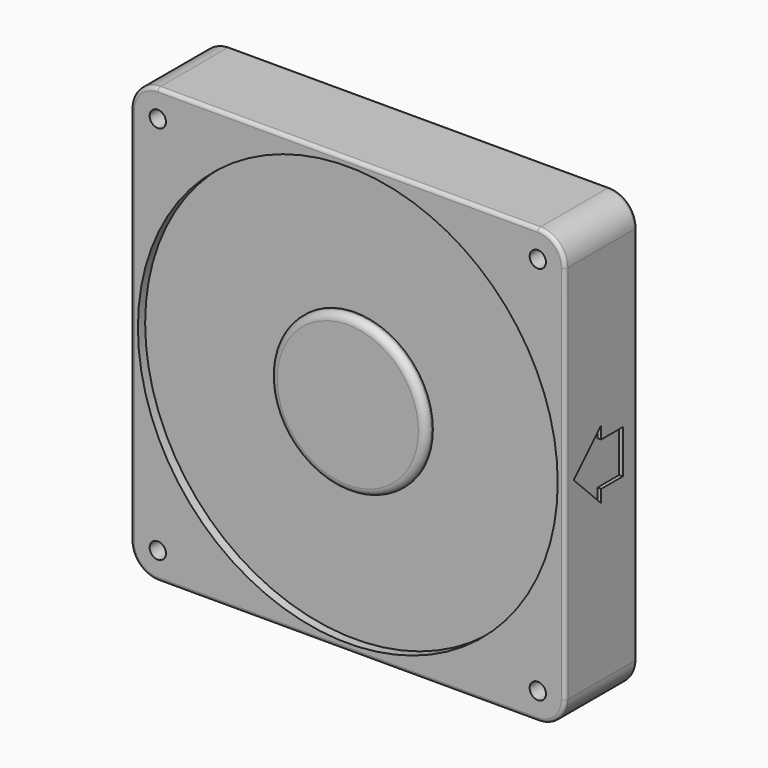
from build123d import *

# Parameters (mm, degrees)
F0_R      = 58
F1_DEPTH  = 12.5
F0_R_2    = 21.5
F2_DEPTH  = 10
F3_R      = 2
F4_R      = 1
F6_D      = 4.5
F8_DEPTH  = 1
F10_DEPTH = 1


with BuildPart() as f1:
    # F0 (on Front) → F1 (new body, symmetric)
    with BuildSketch(Plane.XZ):
        with BuildLine():
            Line((52.5, 60), (-52.5, 60))
            ThreePointArc((-52.5, 60), (-57.8033008589, 57.8033008589), (-60, 52.5))
            Line((-60, 52.5), (-60, -52.5))
            ThreePointArc((-60, -52.5), (-57.8033008589, -57.8033008589), (-52.5, -60))
            Line((-52.5, -60), (52.5, -60))
            ThreePointArc((52.5, -60), (57.8033008589, -57.8033008589), (60, -52.5))
            Line((60, -52.5), (60, 52.5))
            ThreePointArc((60, 52.5), (57.8033008589, 57.8033008589), (52.5, 60))
        make_face()
        Circle(F0_R, mode=Mode.SUBTRACT)
    extrude(amount=F1_DEPTH, both=True)

    # F4
    f4_edges = [f1.edges().sort_by_distance(p)[0] for p in [
        (-60, -12.5, 0),
        (-57.803301, -12.5, -57.803301),
        (0, -12.5, -60),
        (57.803301, -12.5, -57.803301),
        (60, -12.5, 0),
        (57.803301, -12.5, 57.803301),
        (0, -12.5, 60),
        (-57.803301, -12.5, 57.803301),
        (-57.803301, 12.5, -57.803301),
        (0, 12.5, -60),
        (57.803301, 12.5, -57.803301),
        (-60, 12.5, 0),
        (60, 12.5, 0),
        (57.803301, 12.5, 57.803301),
        (0, 12.5, 60),
        (-57.803301, 12.5, 57.803301),
    ]]
    fillet(f4_edges, radius=F4_R)

    # F6 (through all)
    with Locations(Plane.XZ.offset(12.5)):
        with Locations((-52.5, 52.5), (52.5, 52.5), (52.5, -52.5), (-52.5, -52.5)):
            Hole(F6_D / 2)

    # F7 (on face) → F8 (cut)
    with BuildSketch(Plane(origin=(-60, 0, 0), x_dir=(0, -1, 0), z_dir=(-1, 0, 0))):
        Polygon((0, -9.5), (9.5, 0), (0, 9.5), (0, 6), (-7.5, 6), (-7.5, 0), (-7.5, -6), (0, -6), align=None)
    extrude(amount=-F8_DEPTH, mode=Mode.SUBTRACT)

    # F9 (on face) → F10 (cut)
    with BuildSketch(Plane.YZ.offset(60)):
        Polygon((0, 9.5), (-9.5, 0), (0, -9.5), (0, -6), (7.5, -6), (7.5, 0), (7.5, 6), (0, 6), align=None)
    extrude(amount=-F10_DEPTH, mode=Mode.SUBTRACT)


with BuildPart() as f1b:
    # F0 (on Front) → F1, piece 2 (new body, symmetric)
    with BuildSketch(Plane.XZ):
        Circle(F0_R_2)
    extrude(amount=F1_DEPTH, both=True)

    # F0 (on Front) → F2 (join, symmetric)
    with BuildSketch(Plane.XZ):
        Circle(F0_R)
        Circle(F0_R_2, mode=Mode.SUBTRACT)
    extrude(amount=F2_DEPTH, both=True)

    # F3
    f3_edges = [f1b.edges().sort_by_distance(p)[0] for p in [
        (-21.5, -12.5, 0),
        (-21.5, 12.5, 0),
    ]]
    fillet(f3_edges, radius=F3_R)


solid = Compound([f1.part, f1b.part])
